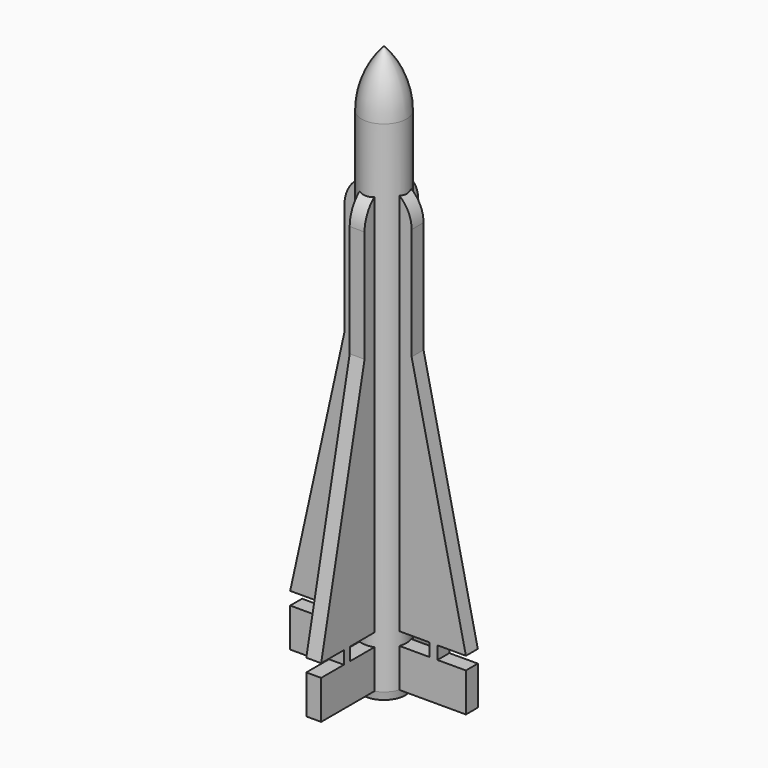
from build123d import *

# Parameters (mm, degrees)
F2_W     = 0.2083333333
F2_H     = 0.3472222222
F3_DEPTH = 0.2
F4_COUNT = 4


# Not quite as in the source:
# - a feature names something its author has since deleted; it is built from what else it names


with BuildPart() as f1:
    # F0 (on Front) → F1 (revolve)
    with BuildSketch(Plane.XZ):
        with BuildLine():
            Line((0, 15.1736111111), (0, 0))
            Line((0, 0), (0.5729166667, 0))
            Line((0.5729166667, 0), (0.6076388889, 0.2083333333))
            Line((0.6076388889, 0.2083333333), (0.6076388889, 13.6458333333))
            ThreePointArc((0.6076388889, 13.6458333333), (0.4501544638, 14.4679236504), (0, 15.1736111111))
        make_face()
    revolve(axis=Axis((0, 0, 7.5868055556), (0, 0, 1)))

    # F2 (on Front) → F3 (join, symmetric)
    with BuildSketch(Plane.XZ):
        with BuildLine():
            Line((0, 12.1101081763), (0, 0.2083333333))
            Line((0, 0.2083333333), (0.6076388889, 0.2083333333))
            Line((0.6076388889, 0.2083333333), (2.3611111111, 0.2083333333))
            Line((2.3611111111, 0.2083333333), (2.3611111111, 1.25))
            Line((2.3611111111, 1.25), (1.5972222222, 1.25))
            Line((1.5972222222, 1.25), (1.3888888889, 1.25))
            Line((1.3888888889, 1.25), (0.4, 1.25))
            Line((0.4, 1.25), (0.4, 1.5972222222))
            Line((0.4, 1.5972222222), (1.3888888889, 1.5972222222))
            Line((1.3888888889, 1.5972222222), (1.5972222222, 1.5972222222))
            Line((1.5972222222, 1.5972222222), (2.3611111111, 1.5972222222))
            Line((2.3611111111, 1.5972222222), (0.9027777778, 8.1944444444))
            Line((0.9027777778, 8.1944444444), (0.9027777778, 11.2073303985))
            ThreePointArc((0.9027777778, 11.2073303985), (0.6383602886, 11.8456906871), (0, 12.1101081763))
        make_face()
        with Locations((1.4930555556, 1.4236111111)):
            Rectangle(F2_W, F2_H)
    extrude(amount=F3_DEPTH, both=True)

    # F4: F1 ×4 about axis
    f4_axis = Axis((0, 0, 0.2083333333), (0, 0, 1))


with BuildPart() as f1_1:
    add(f1.part)
    for i in range(1, F4_COUNT):
        add(f1.part.rotate(f4_axis, i * 360 / F4_COUNT))


solid = f1_1.part
